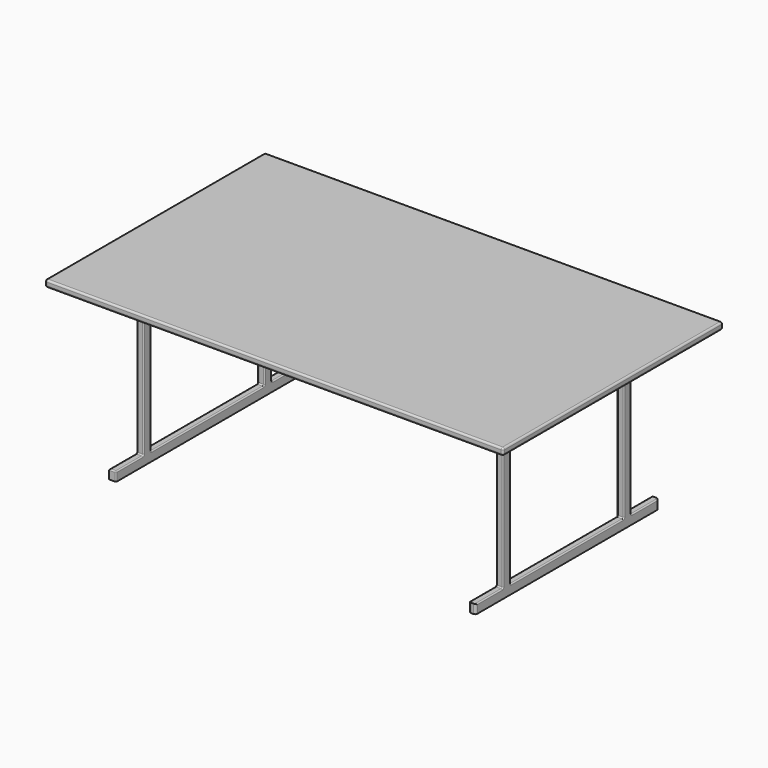
from build123d import *

# Parameters (mm, degrees)
F0_W        = 1200
F0_H        = 30
F1_DEPTH    = 1000
F3_START    = 770
F2_W        = 40
F2_H        = 605
F2_H_2      = 30
F2_W_2      = 150
F2_H_3      = 40
F2_W_3      = 620
F2_R        = 7
F3_DEPTH    = 30
F4_START    = -770
F2_R_2      = 1.5
F4_DEPTH    = 30
F5_DEPTH    = 770
F6_R        = 8
F7_F1_R     = 5
F7_F2_R     = 5
F7_2_F1_R   = 5
F7_2_F2_R   = 5
F8_R        = 5
F8_2_R      = 5
F8_3_R      = 5
F9_T1_DEPTH = 85


# Not quite as in the source:
# - a fillet or chamfer that OpenCascade refuses, or shapes differently, is made with other operations: its cross-section is extruded or revolved along the edge and cut away or added


with BuildPart() as f1:
    # F0 (on Right) → F1 (new body, symmetric)
    with BuildSketch(Plane.YZ):
        Rectangle(F0_W, F0_H)
    extrude(amount=F1_DEPTH, both=True)

    # F6
    f6_edges = [f1.edges().sort_by_distance(p)[0] for p in [
        (0, 600, 15),
        (-1000, 0, 15),
        (0, -600, 15),
        (1000, 0, 15),
        (1000, -600, 0),
        (-1000, 0, -15),
        (0, 600, -15),
        (1000, 0, -15),
        (0, -600, -15),
        (-1000, -600, 0),
        (1000, 600, 0),
        (-1000, 600, 0),
    ]]
    fillet(f6_edges, radius=F6_R)


with BuildPart() as f3:
    # F2 (on Right) → F3 (new body)
    with BuildSketch(Plane.YZ.offset(F3_START)):
        Polygon((500, -690), (350, -690), (310, -690), (-310, -690), (-350, -690), (-500, -690), (-500, -730), (500, -730), align=None)
        with Locations((330, -387.5)):
            Rectangle(F2_W, F2_H)
        with Locations((-330, -387.5)):
            Rectangle(F2_W, F2_H)
        with Locations((-330, -70)):
            Rectangle(F2_W, F2_H_2)
        with Locations((330, -70)):
            Rectangle(F2_W, F2_H_2)
        with Locations((425, -35)):
            Rectangle(F2_W_2, F2_H_3)
        with Locations((0, -35)):
            Rectangle(F2_W_3, F2_H_3)
        with Locations((-425, -35)):
            Rectangle(F2_W_2, F2_H_3)
        with Locations((330, -35)):
            Rectangle(F2_W, F2_H_3)
        with Locations((330, -35)):
            Circle(F2_R, mode=Mode.SUBTRACT)
        with Locations((-330, -35)):
            Rectangle(F2_W, F2_H_3)
        with Locations((-330, -35)):
            Circle(F2_R, mode=Mode.SUBTRACT)
    extrude(amount=F3_DEPTH)

    # F7: fillet of radius 5 on 11 edges, made by hand

    # F7_f1
    f7_f1_edges = [f3.edges().sort_by_distance(p)[0] for p in [
        (785, 310, -55),
        (785, 350, -55),
        (785, -310, -55),
        (785, -350, -55),
        (785, -350, -690),
        (785, -310, -690),
        (785, 350, -690),
        (785, 310, -690),
    ]]
    fillet(f7_f1_edges, radius=F7_F1_R)

    # F7_f2
    f7_f2_edges = [f3.edges().sort_by_distance(p)[0] for p in [
        (800, 0, -55),
        (800, 350, -372.5),
        (800, -427.5, -55),
        (800, -351.4644660941, -56.4644660941),
        (800, 351.4644660941, -688.5355339059),
        (800, 351.4644660941, -56.4644660941),
        (800, -308.5355339059, -56.4644660941),
        (800, 308.5355339059, -56.4644660941),
    ]]
    fillet(f7_f2_edges, radius=F7_F2_R)

    # F8
    f8_edges = [f3.edges().sort_by_distance(p)[0] for p in [
        (770, 427.5, -690),
        (770, 0, -690),
        (770, -427.5, -690),
        (770, -427.5, -55),
        (770, -351.464466, -56.464466),
        (770, -350, -372.5),
        (770, -351.464466, -688.535534),
        (770, 427.5, -55),
        (770, 351.464466, -56.464466),
        (770, 350, -372.5),
        (770, 351.464466, -688.535534),
        (770, -310, -372.5),
        (770, -308.535534, -688.535534),
        (770, -308.535534, -56.464466),
        (770, 0, -55),
        (770, 308.535534, -688.535534),
        (770, 308.535534, -56.464466),
        (770, 310, -372.5),
    ]]
    fillet(f8_edges, radius=F8_R)

    # F9: fillet of radius 10 on 4 edges, made by hand

    # F9_s2 → F9_t1 (cut)
    with BuildSketch(Plane.XY.offset(-755)):
        with BuildLine():
            ThreePointArc((800, 490), (797.0710678119, 497.0710678119), (790, 500))
            Line((790, 500), (800, 500))
            Line((800, 500), (800, 490))
        make_face()
        with BuildLine():
            ThreePointArc((770, 490), (772.9289321881, 497.0710678119), (780, 500))
            Line((780, 500), (770, 500))
            Line((770, 500), (770, 490))
        make_face()
        with BuildLine():
            ThreePointArc((770, -490), (772.9289321881, -497.0710678119), (780, -500))
            Line((780, -500), (770, -500))
            Line((770, -500), (770, -490))
        make_face()
        with BuildLine():
            ThreePointArc((800, -490), (797.0710678119, -497.0710678119), (790, -500))
            Line((790, -500), (800, -500))
            Line((800, -500), (800, -490))
        make_face()
    extrude(amount=F9_T1_DEPTH, mode=Mode.SUBTRACT)


with BuildPart() as f4:
    # F2 (on Right) → F4 (new body)
    with BuildSketch(Plane.YZ.offset(F4_START)):
        with Locations((425, -35)):
            Rectangle(F2_W_2, F2_H_3)
        with Locations((0, -35)):
            Rectangle(F2_W_3, F2_H_3)
        with Locations((-425, -35)):
            Rectangle(F2_W_2, F2_H_3)
        with Locations((330, -70)):
            Rectangle(F2_W, F2_H_2)
        with Locations((330, -387.5)):
            Rectangle(F2_W, F2_H)
        Polygon((500, -690), (350, -690), (310, -690), (-310, -690), (-350, -690), (-500, -690), (-500, -730), (500, -730), align=None)
        with Locations((-330, -387.5)):
            Rectangle(F2_W, F2_H)
        with Locations((-330, -70)):
            Rectangle(F2_W, F2_H_2)
        with Locations((-330, -35)):
            Rectangle(F2_W, F2_H_3)
        with Locations((-330, -35)):
            Circle(F2_R, mode=Mode.SUBTRACT)
        with Locations((330, -35)):
            Rectangle(F2_W, F2_H_3)
        with Locations((330, -35)):
            Circle(F2_R, mode=Mode.SUBTRACT)
        with Locations((330, -35)):
            Circle(F2_R)
        with Locations((330, -35)):
            Circle(F2_R_2, mode=Mode.SUBTRACT)
        with Locations((-330, -35)):
            Circle(F2_R)
        with Locations((-330, -35)):
            Circle(F2_R_2, mode=Mode.SUBTRACT)
    extrude(amount=-F4_DEPTH)

    # F7#2: fillet of radius 5 on 20 edges, made by hand

    # F7_2_f1
    f7_2_f1_edges = [f4.edges().sort_by_distance(p)[0] for p in [
        (-785, -350, -55),
        (-785, -310, -55),
        (-785, 310, -55),
        (-785, 350, -55),
        (-785, -350, -690),
        (-785, -310, -690),
        (-785, 310, -690),
        (-785, 350, -690),
    ]]
    fillet(f7_2_f1_edges, radius=F7_2_F1_R)

    # F7_2_f2
    f7_2_f2_edges = [f4.edges().sort_by_distance(p)[0] for p in [
        (-800, -427.5, -55),
        (-800, 0, -55),
        (-800, 427.5, -55),
        (-800, -427.5, -690),
        (-800, 500, -710),
        (-785, 500, -690),
        (-785, -500, -690),
        (-770, -500, -710),
        (-770, -427.5, -690),
        (-770, -310, -372.5),
        (-770, 427.5, -690),
        (-770, 500, -710),
        (-770, 351.4644660941, -688.5355339059),
        (-770, -308.5355339059, -688.5355339059),
        (-770, -308.5355339059, -56.4644660941),
        (-770, -351.4644660941, -688.5355339059),
        (-800, -351.4644660941, -688.5355339059),
        (-800, 351.4644660941, -56.4644660941),
        (-800, -308.5355339059, -56.4644660941),
        (-800, 308.5355339059, -56.4644660941),
        (-800, -351.4644660941, -56.4644660941),
    ]]
    fillet(f7_2_f2_edges, radius=F7_2_F2_R)


with BuildPart() as f5:
    # F2 (on Right) → F5 (new body, symmetric)
    with BuildSketch(Plane.YZ):
        with Locations((-330, -70)):
            Rectangle(F2_W, F2_H_2)
        with Locations((-330, -35)):
            Rectangle(F2_W, F2_H_3)
        with Locations((-330, -35)):
            Circle(F2_R, mode=Mode.SUBTRACT)
    extrude(amount=F5_DEPTH, both=True)

    # F8#2
    f8_2_edges = [f5.edges().sort_by_distance(p)[0] for p in [
        (0, -350, -85),
        (0, -310, -85),
    ]]
    fillet(f8_2_edges, radius=F8_2_R)


with BuildPart() as f5b:
    # F2 (on Right) → F5, piece 2 (new body, symmetric)
    with BuildSketch(Plane.YZ):
        with Locations((330, -70)):
            Rectangle(F2_W, F2_H_2)
        with Locations((330, -35)):
            Rectangle(F2_W, F2_H_3)
        with Locations((330, -35)):
            Circle(F2_R, mode=Mode.SUBTRACT)
    extrude(amount=F5_DEPTH, both=True)

    # F8#3
    f8_3_edges = [f5b.edges().sort_by_distance(p)[0] for p in [
        (0, 350, -85),
        (0, 310, -85),
    ]]
    fillet(f8_3_edges, radius=F8_3_R)


solid = Compound([f1.part, f3.part, f4.part, f5.part, f5b.part])
